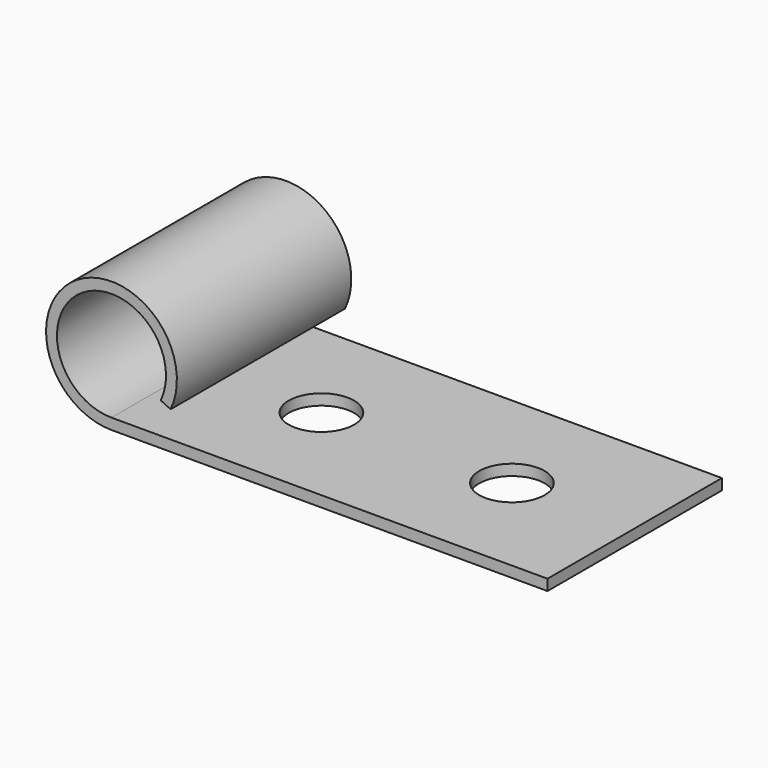
from build123d import *

# Parameters (mm, degrees)
F1_DEPTH = 10
F3_D     = 3


# Not quite as in the source:
# - ends of sketch curves that miss each other by under 0.0002 mm in the source are joined


with BuildPart() as f1:
    # F0 (on Front) → F1 (new body)
    with BuildSketch(Plane.XZ):
        with BuildLine():
            ThreePointArc((13.5271953943, 27.6566442743), (9.210189973, 31.473808666), (10.8152050392, 25.9392620325))
            Line((10.8152050392, 25.9392620325), (30.8152050392, 25.9392620325))
            Line((30.8152050392, 25.9392620325), (30.8152050392, 26.439262554))
            Line((30.8152050392, 26.439262554), (10.8152050392, 26.439262554))
            ThreePointArc((10.8152050392, 26.439262554), (9.4776924841, 31.0513842271), (13.0751970018, 27.8704139006))
            Line((13.0751970018, 27.8704139006), (13.5271953943, 27.6566442743))
        make_face()
    extrude(amount=F1_DEPTH)

    # F3 (through all)
    with Locations(Plane.XY.offset(26.439262554)):
        with Locations((16.4454622901, -5), (25.1849477884, -5)):
            Hole(F3_D / 2)


solid = f1.part
